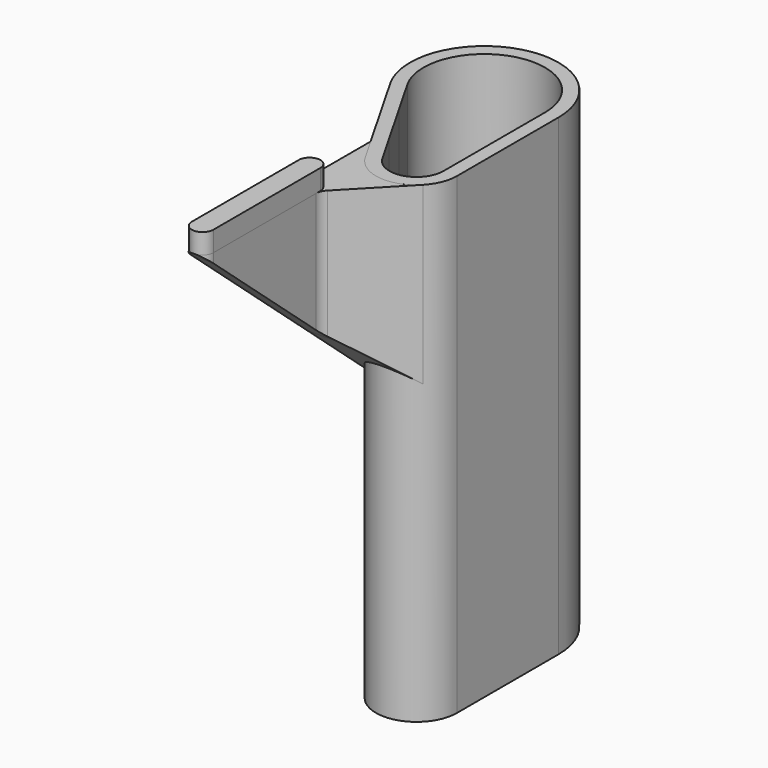
from build123d import *

# Parameters (mm, degrees)
F0_R      = 5.5
F0_R_2    = 4.5
F1_DEPTH  = 35
F3_DEPTH  = 1.5
F5_DEPTH  = 35
F7_DEPTH  = 35
F9_DEPTH  = 35.001
F11_DEPTH = 15
F13_DEPTH = 25
F14_R     = 1


# Not quite as in the source:
# - ends of sketch curves that miss each other by under 0.0002 mm in the source are joined


with BuildPart() as f1:
    # F0 (on Top) → F1 (new body)
    with BuildSketch(Plane.XY):
        Circle(F0_R)
        Circle(F0_R_2, mode=Mode.SUBTRACT)
    extrude(amount=F1_DEPTH)

    # F6 (on face) → F7 (join)
    with BuildSketch(Plane.XY.offset(35)):
        with BuildLine():
            Line((-0.5, -9.4), (-0.5, -8.1848935982))
            Line((-0.5, -8.1848935982), (-2.3345095585, -4.9799663775))
            ThreePointArc((-2.3345095585, -4.9799663775), (-3.7273838867, -4.0443305207), (-4.773332625, -2.7322693226))
            Line((-4.773332625, -2.7322693226), (-0.1036359901, -10.8903286733))
            ThreePointArc((-0.1036359901, -10.8903286733), (-0.3992160983, -10.1710680876), (-0.5, -9.4))
        make_face()
        with BuildLine():
            ThreePointArc((5.5, 0), (5.2440441901, -1.6583125558), (4.4999998063, -3.1622779358))
            Line((4.4999998063, -3.1622779358), (4.4999998063, -9.4))
            ThreePointArc((4.4999998063, -9.4), (3.0140452866, -11.3328106364), (0.764242669, -10.3935524328))
            Line((0.764242669, -10.3935524328), (-0.5, -8.1848935982))
            Line((-0.5, -8.1848935982), (-0.5, -9.4))
            ThreePointArc((-0.5, -9.4), (-0.3992160983, -10.1710680876), (-0.1036359901, -10.8903286733))
            ThreePointArc((-0.1036359901, -10.8903286733), (3.2710679908, -12.2992160015), (5.4999998063, -9.4))
            Line((5.4999998063, -9.4), (5.5, 0))
        make_face()
    extrude(amount=-F7_DEPTH)

    # F8 (on face) → F9 (cut, through all)
    with BuildSketch(Plane.XY.offset(35)):
        with BuildLine():
            Line((-3.9054539659, -2.2354930822), (-2.3345095585, -4.9799663775))
            ThreePointArc((-2.3345095585, -4.9799663775), (1.4136247101, -5.3152295509), (4.4999998063, -3.1622779358))
            Line((4.4999998063, -3.1622779358), (4.5, 0))
            ThreePointArc((4.5, 0), (1.1566021688, -4.3488241426), (-3.9054539659, -2.2354930822))
        make_face()
    extrude(amount=-F9_DEPTH, mode=Mode.SUBTRACT)


with BuildPart() as f1b:
    # F0 (on Top) → F1, piece 2 (new body)
    with BuildSketch(Plane.XY):
        with BuildLine():
            Line((0.5, -25.7), (0.5, -15.8))
            ThreePointArc((0.5, -15.8), (-0.3, -15), (-1.1, -15.8))
            Line((-1.1, -15.8), (-1.1, -25.7))
            ThreePointArc((-1.1, -25.7), (-0.3, -26.5), (0.5, -25.7))
        make_face()
    extrude(amount=F1_DEPTH)

    # F4 (on face) → F5 (cut)
    with BuildSketch(Plane(origin=(0, 0, 0), x_dir=(1, 0, 0), z_dir=(0, 0, -1))):
        with BuildLine():
            Line((-1.1, 25.7), (-1.1, 15.8))
            ThreePointArc((-1.1, 15.8), (-0.3, 15), (0.5, 15.8))
            Line((0.5, 15.8), (0.5, 25.7))
            ThreePointArc((0.5, 25.7), (-0.3, 26.5), (-1.1, 25.7))
        make_face()
    extrude(amount=-F5_DEPTH, mode=Mode.SUBTRACT)


with BuildPart() as f3:
    # F2 (on face) → F3 (new body)
    with BuildSketch(Plane.XY.offset(35)):
        with BuildLine():
            Line((0.5, -25.7), (0.5, -15.8))
            ThreePointArc((0.5, -15.8), (-0.3, -15), (-1.1, -15.8))
            Line((-1.1, -15.8), (-1.1, -25.7))
            ThreePointArc((-1.1, -25.7), (-0.3, -26.5), (0.5, -25.7))
        make_face()
    extrude(amount=F3_DEPTH)


with BuildPart() as f11:
    # F10 (on face) → F11 (new body)
    with BuildSketch(Plane.XY.offset(35)):
        with BuildLine():
            ThreePointArc((-1.1, -15.8), (-0.3, -15), (0.5, -15.8))
            Line((0.5, -15.8), (4.6604977162, -11.4814054431))
            ThreePointArc((4.6604977162, -11.4814054431), (2.130627765, -12.3771737676), (-0.1036359901, -10.8903286733))
            Line((-0.1036359901, -10.8903286733), (-1.1, -9.1496595542))
            Line((-1.1, -9.1496595542), (-1.1, -15.8))
        make_face()
        with BuildLine():
            ThreePointArc((-1.1, -25.7), (-0.3, -26.5), (0.5, -25.7))
            Line((0.5, -25.7), (0.5, -15.8))
            ThreePointArc((0.5, -15.8), (-0.3, -15), (-1.1, -15.8))
            Line((-1.1, -15.8), (-1.1, -25.7))
        make_face()
    extrude(amount=-F11_DEPTH)

    # F12 (on face) → F13 (cut)
    with BuildSketch(Plane(origin=(-1.1, 0, 0), x_dir=(0, -1, 0), z_dir=(-1, 0, 0))):
        Polygon((15, 20), (15, 25.0578319752), (9.1496595542, 20), align=None)
        Polygon((25.7, 34.30837092), (15, 25.0578319752), (15, 20), (25.7, 20), align=None)
        Polygon((26.5, 20), (26.5, 35), (25.7, 34.30837092), (25.7, 20), align=None)
    extrude(amount=-F13_DEPTH, mode=Mode.SUBTRACT)

    # F14
    f14_edges = [f11.edges().sort_by_distance(p)[0] for p in [
        (0.5, -15.8, 30.374731),
    ]]
    fillet(f14_edges, radius=F14_R)


solid = Compound([f1.part, f3.part, f11.part])
